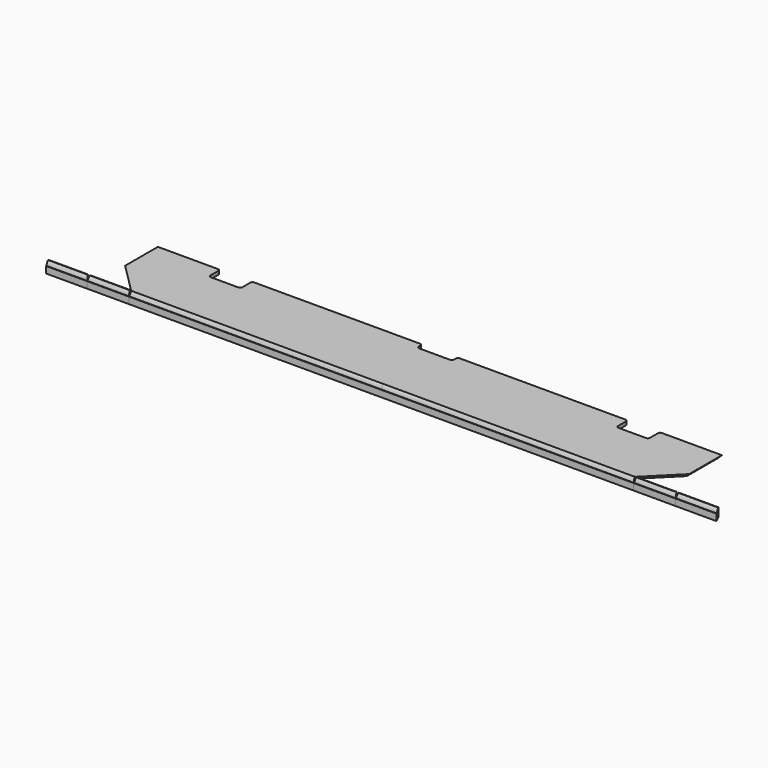
from build123d import *

# Parameters (mm, degrees)
F3_DEPTH      = 10.16
F4_W          = 2032
F4_H          = 7.9375
F5_DEPTH      = 57.15
F7_DEPTH      = 1016.001
F7_DEPTH_BACK = 1016.001
F9_DEPTH      = 2032.0010001
F10_W         = 49.9748663003
F10_H         = 7.9375
F11_DEPTH     = 31.7510001
F12_W         = 92.075
F12_H         = 41.275
F12_W_2       = 101.6
F12_H_2       = 19.05
F13_DEPTH     = 31.7510001
F14_R         = 6.35
F15_SIZE      = 10.15999


# Not quite as in the source:
# - a variable given as a bare number and used for a length is read in inches; the dataset says mm whatever the document's units were
# - a fillet or chamfer is up to 0.001 mm smaller than in the source, because OpenCascade refuses the exact size


with BuildPart() as f3:
    # F2 (on Top) → F3 (new body)
    with BuildSketch(Plane.XY):
        Polygon((812.8, 0), (-812.8, 0), (-812.8, -117.8875668498), (-727.4875668498, -203.2), (727.4875668498, -203.2), (812.8, -117.8875668498), align=None)
    extrude(amount=-F3_DEPTH)

    # F12 (on face) → F13 (cut, through all)
    with BuildSketch(Plane.XY):
        with Locations((-587.375, -20.6375)):
            Rectangle(F12_W, F12_H)
        with Locations((0, -9.525)):
            Rectangle(F12_W_2, F12_H_2)
        with Locations((587.375, -20.6375)):
            Rectangle(F12_W, F12_H)
    extrude(amount=-F13_DEPTH, mode=Mode.SUBTRACT)

    # F14
    f14_edges = [f3.edges().sort_by_distance(p)[0] for p in [
        (-633.4125, 0, -5.08),
        (-633.4125, -41.275, -5.08),
        (-541.3375, -41.275, -5.08),
        (-541.3375, 0, -5.08),
        (-50.8, -19.05, -5.08),
        (-50.8, 0, -5.08),
        (50.8, 0, -5.08),
        (50.8, -19.05, -5.08),
        (633.4125, -41.275, -5.08),
        (633.4125, 0, -5.08),
        (541.3375, -41.275, -5.08),
        (541.3375, 0, -5.08),
    ]]
    fillet(f14_edges, radius=F14_R)

    # F15 (size 10.16 in the source; OpenCascade refuses exactly that, so slightly less here)
    f15_edges = [f3.edges().sort_by_distance(p)[0] for p in [
        (770.143783, -160.543783, -10.16),
        (812.8, -58.943783, -10.16),
        (-812.8, -58.943783, -10.16),
        (-770.143783, -160.543783, -10.16),
        (0, -203.2, -10.16),
    ]]
    chamfer(f15_edges, length=F15_SIZE)


with BuildPart() as f5:
    # F4 (on face) → F5 (new body)
    with BuildSketch(Plane.XY):
        with Locations((0, -207.16875)):
            Rectangle(F4_W, F4_H)
    extrude(amount=-F5_DEPTH)

    # F6 (on Right) → F7 (cut, two sides)
    with BuildSketch(Plane.YZ) as f7_sk:
        with BuildLine():
            Line((-211.1375, -12.7), (-209.6375, -12.7))
            add(Edge.make_bspline(
                [(-204.7, 0), (-204.7, -0.2210937751), (-204.7812100527, -1.0944146655), (-208.0488035194, -4.6634409415), (-209.5721225282, -10.9497164159), (-209.6375, -12.7)],
                knots=[0, 0, 0, 0, 0.1542509364, 0.52215781, 1, 1, 1, 1], degree=3))
            Line((-204.7, 0), (-211.1375, 0))
            Line((-211.1375, 0), (-211.1375, -12.7))
        make_face()
    extrude(amount=-F7_DEPTH, mode=Mode.SUBTRACT)
    extrude(f7_sk.sketch, amount=F7_DEPTH_BACK, mode=Mode.SUBTRACT)

    # F8 (on face) → F9 (cut, through all)
    with BuildSketch(Plane.YZ.offset(1016)):
        Polygon((-203.2, -23.8125), (-211.1375, -31.75), (-211.1375, -57.15), (-203.2, -57.15), align=None)
    extrude(amount=-F9_DEPTH, mode=Mode.SUBTRACT)

    # F10 (on face) → F11 (cut, through all)
    with BuildSketch(Plane.XY):
        Polygon((-727.4875668498, -211.1375), (-724.1997466985, -203.2), (-730.7753870012, -203.2), align=None)
        Polygon((-848.1375668498, -211.1375), (-844.8497466985, -203.2), (-851.4253870012, -203.2), align=None)
        Polygon((730.7753870012, -203.2), (724.1997466985, -203.2), (727.4875668498, -211.1375), align=None)
        Polygon((851.4253870012, -203.2), (844.8497466985, -203.2), (848.1375668498, -211.1375), align=None)
        with Locations((-991.0125668498, -207.16875)):
            Rectangle(F10_W, F10_H)
        with Locations((991.0125668498, -207.16875)):
            Rectangle(F10_W, F10_H)
    extrude(amount=-F11_DEPTH, mode=Mode.SUBTRACT)


solid = Compound([f3.part, f5.part])
